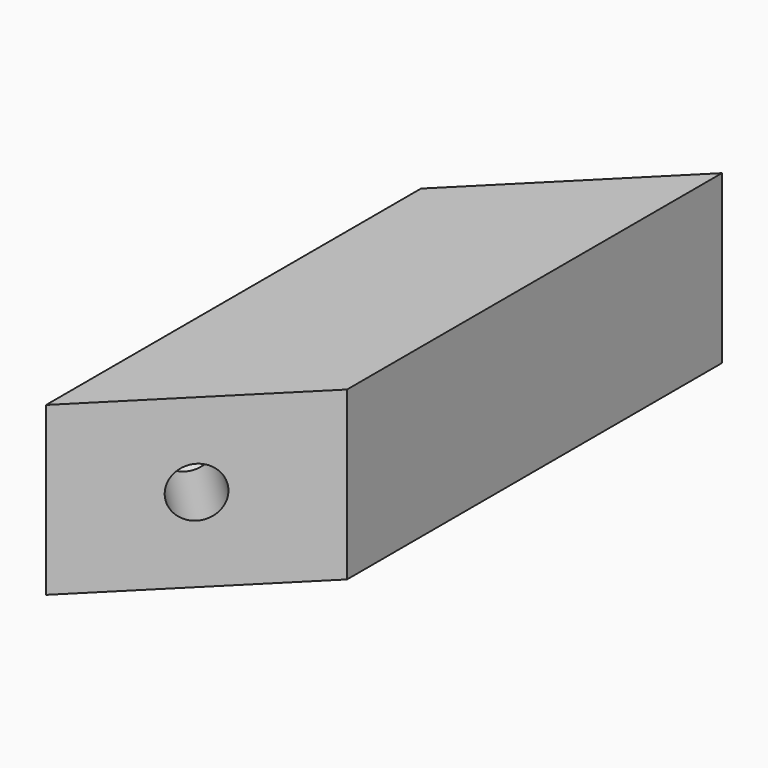
from build123d import *

# Parameters (mm, degrees)
F0_W           = 12.7
F0_H           = 48.29048
F1_DEPTH       = 12.7
F2_SIZE2       = 12.69999
F2_SIZE        = 12.69999
F3_SIZE2       = 12.69999
F3_SIZE        = 12.69999
F6_D           = 3.81
F6_DEPTH       = 6.35
F6_TIP         = 1.1446394792
F6_ON_F4_D     = 3.81
F6_ON_F4_DEPTH = 6.35
F6_ON_F4_TIP   = 1.1446394792


# Not quite as in the source:
# - a fillet or chamfer is up to 0.001 mm smaller than in the source, because OpenCascade refuses the exact size


with BuildPart() as f1:
    # F0 (on Top) → F1 (new body)
    with BuildSketch(Plane.XY):
        with Locations((1.3377478731, 0)):
            Rectangle(F0_W, F0_H)
    extrude(amount=F1_DEPTH)

    # F2 (size 12.7 and 12.7 in the source; OpenCascade refuses exactly that, so slightly less here)
    f2_edges = [f1.edges().sort_by_distance(p)[0] for p in [
        (7.687748, -24.14524, 6.35),
    ]]
    chamfer(f2_edges, length=F2_SIZE, length2=F2_SIZE2)

    # F3 (size 12.7 and 12.7 in the source; OpenCascade refuses exactly that, so slightly less here)
    f3_edges = [f1.edges().sort_by_distance(p)[0] for p in [
        (-5.012252, 24.14524, 6.35),
    ]]
    chamfer(f3_edges, length=F3_SIZE, length2=F3_SIZE2)

    # F6
    with Locations(Plane(origin=(9.5664939365, -9.5664939365, 0), x_dir=(0.7071067812, 0.7071067812, 0), z_dir=(0.7071067812, -0.7071067812, 0))):
        with Locations((-11.6371181632, 6.35)):
            Hole(F6_D / 2, depth=F6_DEPTH)
            with Locations((0, 0, -(F6_DEPTH + F6_TIP / 2))):  # 118° drill point
                Cone(0, F6_D / 2, F6_TIP, mode=Mode.SUBTRACT)

    # F6 on F4
    with Locations(Plane(origin=(-8.2287460635, 8.2287460635, 0), x_dir=(-0.7071067812, -0.7071067812, 0), z_dir=(-0.7071067812, 0.7071067812, 0))):
        with Locations((-13.5289793484, 6.35)):
            Hole(F6_ON_F4_D / 2, depth=F6_ON_F4_DEPTH)
            with Locations((0, 0, -(F6_ON_F4_DEPTH + F6_ON_F4_TIP / 2))):  # 118° drill point
                Cone(0, F6_ON_F4_D / 2, F6_ON_F4_TIP, mode=Mode.SUBTRACT)


solid = f1.part
